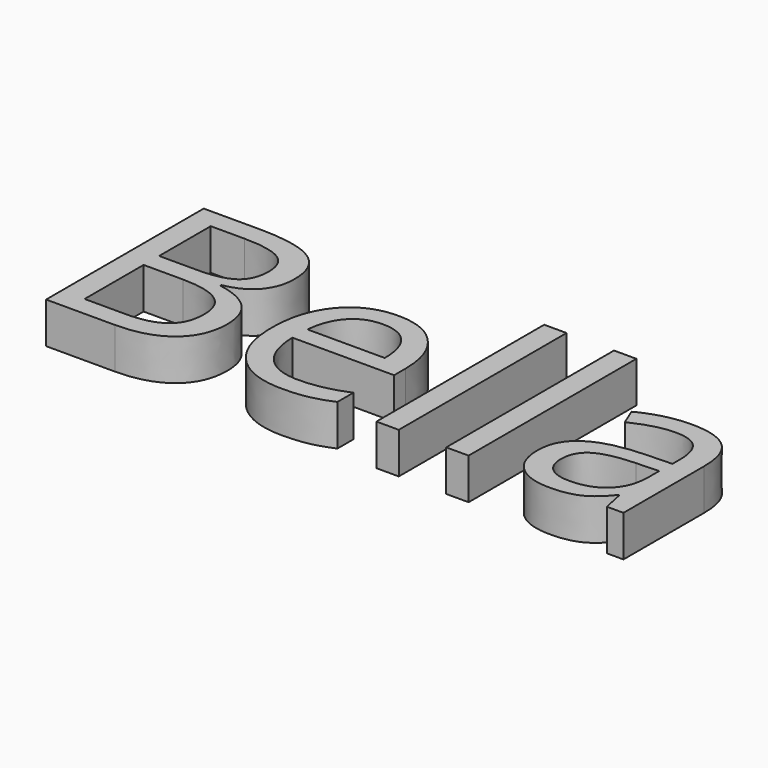
from build123d import *

# Parameters (mm, degrees)
F0_TEXT_SIZE = 170.7608889168
F1_DEPTH     = 25.4


# Not quite as in the source:
# - Text() gives the source's letters only with a copy of the font that has no kerning and outlines rounded to 1/6400 em; it was checked with that copy


with BuildPart() as f1:
    # F0 (on Top) → F1 (new body)
    with BuildSketch(Plane.XY):
        with Locations((-149.9363910407, -58.2626857795)):
            Text('Bella', F0_TEXT_SIZE, font='Open Sans', text_align=(TextAlign.LEFT, TextAlign.BOTTOM))
    extrude(amount=F1_DEPTH)


solid = f1.part
